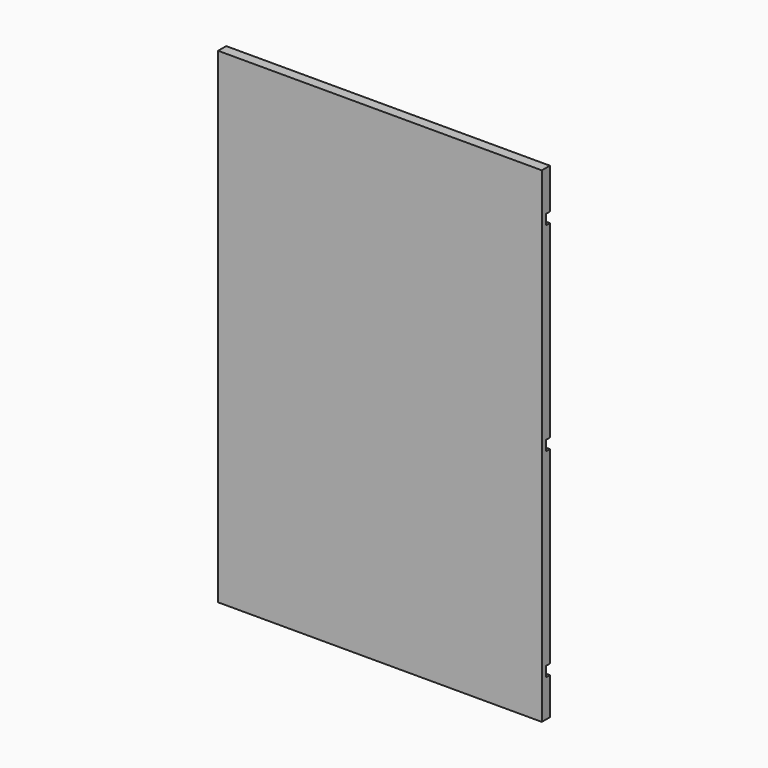
from build123d import *

# Parameters (mm, degrees)
F0_W     = 609.6
F0_H     = 914.4
F1_DEPTH = 19.05
F2_W     = 609.6
F2_H     = 19.05
F3_DEPTH = 9.525


# Not quite as in the source:
# - a length typed as a fraction of an inch, garbled in the dataset ("3 / 203.2 mm" for 3/8 in), is restored


with BuildPart() as f1:
    # F0 (on Front) → F1 (new body)
    with BuildSketch(Plane.XZ):
        with Locations((304.8, 457.2)):
            Rectangle(F0_W, F0_H)
    extrude(amount=F1_DEPTH)

    # F2 (on face) → F3 (cut)
    with BuildSketch(Plane(origin=(0, 0, 0), x_dir=(-1, 0, 0), z_dir=(0, 1, 0))):
        with Locations((-304.8, 79.375)):
            Rectangle(F2_W, F2_H)
        with Locations((-304.8, 454.025)):
            Rectangle(F2_W, F2_H)
        with Locations((-304.8, 828.675)):
            Rectangle(F2_W, F2_H)
    extrude(amount=-F3_DEPTH, mode=Mode.SUBTRACT)


solid = f1.part
